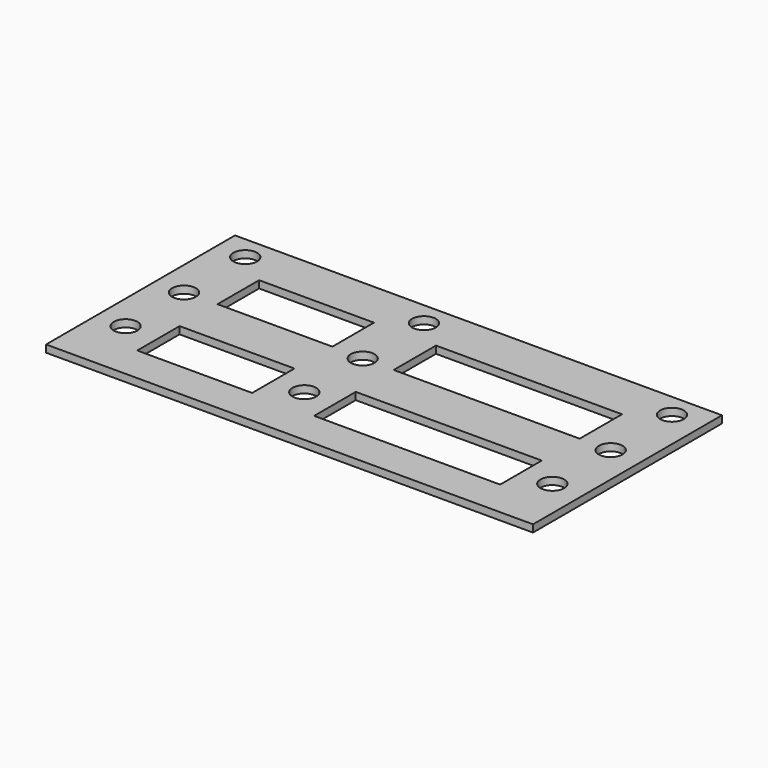
from build123d import *

# Parameters (mm, degrees)
F0_R     = 3.25
F0_W     = 31.5
F0_H     = 13
F0_W_2   = 51
F1_DEPTH = 2
F2_DEPTH = 2


# Not quite as in the source:
# - a feature names something its author has since deleted; it is built from what else it names


with BuildPart() as f1:
    # F0 (on Top) → F1 (new body)
    with BuildSketch(Plane.XY):
        Polygon((-26.2163661122, 15.2858447556), (-43.2163661122, 15.2858447556), (-43.2163661122, -26.4641552444), (-26.2163661122, -26.4641552444), (-26.2163661122, -11.9641552444), (-26.2163661122, 1.0358447556), align=None)
        with Locations((-35.2163661122, -19.2141552444)):
            Circle(F0_R, mode=Mode.SUBTRACT)
        with Locations((-35.2163661122, 0.7858447556)):
            Circle(F0_R, mode=Mode.SUBTRACT)
        Polygon((22.2836338878, 15.2858447556), (5.2836338878, 15.2858447556), (5.2836338878, 1.0358447556), (5.2836338878, -11.9641552444), (5.2836338878, -26.4641552444), (22.2836338878, -26.4641552444), (22.2836338878, -12.2141552444), (22.2836338878, 0.7858447556), align=None)
        with Locations((13.7836338878, -19.2141552444)):
            Circle(F0_R, mode=Mode.SUBTRACT)
        with Locations((13.7836338878, 0.7858447556)):
            Circle(F0_R, mode=Mode.SUBTRACT)
        Polygon((90.2836338878, -26.4641552444), (90.2836338878, 15.2858447556), (73.2836338878, 15.2858447556), (73.2836338878, 0.7858447556), (73.2836338878, -12.2141552444), (73.2836338878, -26.4641552444), align=None)
        with Locations((81.7836338878, -19.2141552444)):
            Circle(F0_R, mode=Mode.SUBTRACT)
        with Locations((81.7836338878, 0.7858447556)):
            Circle(F0_R, mode=Mode.SUBTRACT)
        Polygon((-26.2163661122, -26.4641552444), (-43.2163661122, -26.4641552444), (-43.2163661122, -36.4641552444), (90.2836338878, -36.4641552444), (90.2836338878, -26.4641552444), (73.2836338878, -26.4641552444), (22.2836338878, -26.4641552444), (5.2836338878, -26.4641552444), align=None)
        with Locations((-10.4663661122, -5.4641552444)):
            Rectangle(F0_W, F0_H)
        with Locations((47.7836338878, -5.7141552444)):
            Rectangle(F0_W_2, F0_H)
    extrude(amount=F1_DEPTH)

    # F0 (on Top) → F2 (join)
    with BuildSketch(Plane.XY):
        Polygon((90.2836338878, 28.2858447556), (-43.2163661122, 28.2858447556), (-43.2163661122, 15.2858447556), (-26.2163661122, 15.2858447556), (5.2836338878, 15.2858447556), (22.2836338878, 15.2858447556), (73.2836338878, 15.2858447556), (90.2836338878, 15.2858447556), align=None)
        with Locations((-35.2163661122, 21.7858447556)):
            Circle(F0_R, mode=Mode.SUBTRACT)
        with Locations((13.7836338878, 21.7858447556)):
            Circle(F0_R, mode=Mode.SUBTRACT)
        with Locations((81.7836338878, 21.7858447556)):
            Circle(F0_R, mode=Mode.SUBTRACT)
    extrude(amount=F2_DEPTH)


solid = f1.part
